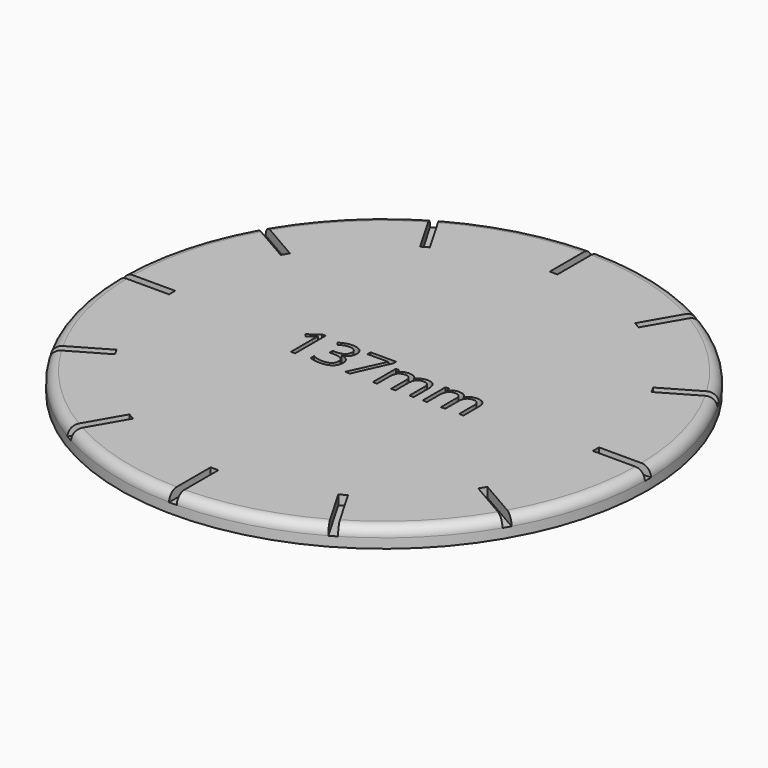
from build123d import *

# Parameters (mm, degrees)
F0_R         = 68.5
F1_DEPTH     = 5
F2_W         = 2
F2_H         = 15
F2_W_2       = 15
F2_H_2       = 2
F3_DEPTH     = 2.5
F4_TEXT_SIZE = 13.888889872
F5_DEPTH     = 2.5
F6_R         = 2.5


# Not quite as in the source:
# - Text() gives the source's letters only with a copy of the font that has no kerning and outlines rounded to 1/6400 em; it was checked with that copy


with BuildPart() as f1:
    # F0 (on Top) → F1 (new body)
    with BuildSketch(Plane.XY):
        Circle(F0_R)
    extrude(amount=F1_DEPTH)

    # F2 (on face) → F3 (cut)
    with BuildSketch(Plane.XY.offset(5)):
        with Locations((0, 62.5)):
            Rectangle(F2_W, F2_H)
        Polygon((-34.1339745962, 61.1217782649), (-35.8660254038, 60.1217782649), (-28.3660254038, 47.1313972081), (-26.6339745962, 48.1313972081), align=None)
        Polygon((-60.1217782649, 35.8660254038), (-61.1217782649, 34.1339745962), (-48.1313972081, 26.6339745962), (-47.1313972081, 28.3660254038), align=None)
        with Locations((-62.5, 0)):
            Rectangle(F2_W_2, F2_H_2)
        Polygon((-61.1217782649, -34.1339745962), (-60.1217782649, -35.8660254038), (-47.1313972081, -28.3660254038), (-48.1313972081, -26.6339745962), align=None)
        Polygon((-35.8660254038, -60.1217782649), (-34.1339745962, -61.1217782649), (-26.6339745962, -48.1313972081), (-28.3660254038, -47.1313972081), align=None)
        with Locations((0, -62.5)):
            Rectangle(F2_W, F2_H)
        Polygon((34.1339745962, -61.1217782649), (35.8660254038, -60.1217782649), (28.3660254038, -47.1313972081), (26.6339745962, -48.1313972081), align=None)
        Polygon((60.1217782649, -35.8660254038), (61.1217782649, -34.1339745962), (48.1313972081, -26.6339745962), (47.1313972081, -28.3660254038), align=None)
        with Locations((62.5, 0)):
            Rectangle(F2_W_2, F2_H_2)
        Polygon((61.1217782649, 34.1339745962), (60.1217782649, 35.8660254038), (47.1313972081, 28.3660254038), (48.1313972081, 26.6339745962), align=None)
        Polygon((35.8660254038, 60.1217782649), (34.1339745962, 61.1217782649), (26.6339745962, 48.1313972081), (28.3660254038, 47.1313972081), align=None)
    extrude(amount=-F3_DEPTH, mode=Mode.SUBTRACT)

    # F4 (on face) → F5 (cut)
    with BuildSketch(Plane.XY.offset(5)):
        with Locations((-23.7285758194, -5.2462602034)):
            Text('137mm', F4_TEXT_SIZE, font='Open Sans', text_align=(TextAlign.LEFT, TextAlign.BOTTOM))
    extrude(amount=-F5_DEPTH, mode=Mode.SUBTRACT)

    # F6
    f6_edges = [f1.edges().sort_by_distance(p)[0] for p in [
        (48.436815, 48.436815, 5),
        (66.165919, 17.729105, 5),
        (66.165919, -17.729105, 5),
        (48.436815, -48.436815, 5),
        (17.729105, -66.165919, 5),
        (-17.729105, -66.165919, 5),
        (-48.436815, -48.436815, 5),
        (-66.165919, -17.729105, 5),
        (-66.165919, 17.729105, 5),
        (-48.436815, 48.436815, 5),
        (-17.729105, 66.165919, 5),
        (17.729105, 66.165919, 5),
    ]]
    fillet(f6_edges, radius=F6_R)


solid = f1.part
